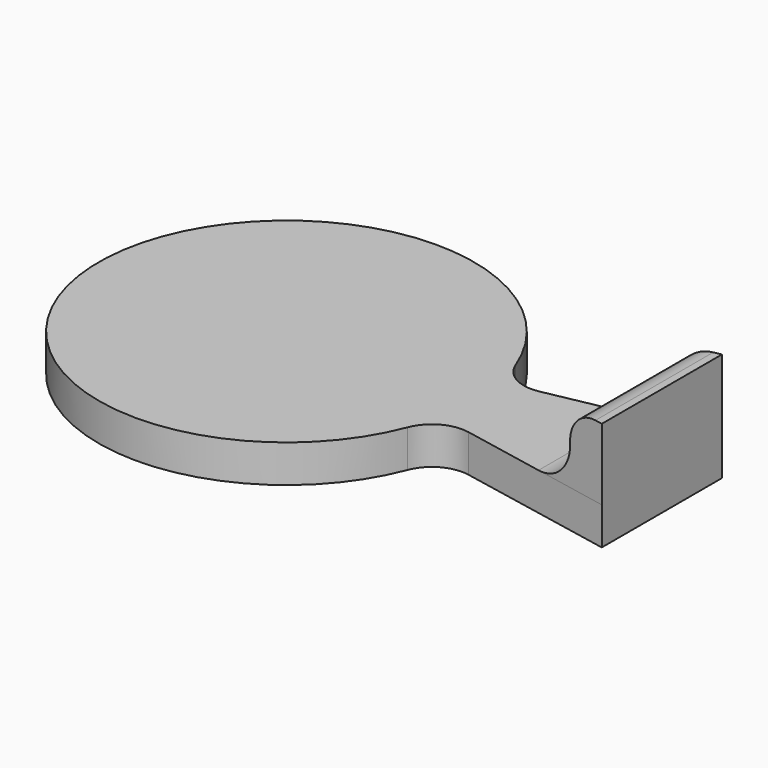
from build123d import *

# Parameters (mm, degrees)
F1_DEPTH = 5
F3_DEPTH = 9.5
F4_R     = 5
F5_R     = 4


# Not quite as in the source:
# - a feature names something its author has since deleted; it is built from what else it names


with BuildPart() as f1:
    # F0 (on Top) → F1 (new body)
    with BuildSketch(Plane.XY):
        with BuildLine():
            Line((50, 10), (24.4948974278, 5))
            ThreePointArc((24.4948974278, 5), (-25, 0), (24.4948974278, -5))
            Line((24.4948974278, -5), (50, -10))
            Line((50, -10), (50, 10))
        make_face()
    extrude(amount=F1_DEPTH)

    # F2 (on face) → F3 (join)
    with BuildSketch(Plane.XY.offset(5)):
        Polygon((50, -10), (50, 10), (45, 9.0198039812), (45, -9.0198039812), align=None)
    extrude(amount=F3_DEPTH)

    # F4
    f4_edges = [f1.edges().sort_by_distance(p)[0] for p in [
        (45, 0, 5),
        (24.494897, -5, 2.5),
        (24.494897, 5, 2.5),
    ]]
    fillet(f4_edges, radius=F4_R)

    # F5
    f5_edges = [f1.edges().sort_by_distance(p)[0] for p in [
        (45, 0, 14.5),
    ]]
    fillet(f5_edges, radius=F5_R)


solid = f1.part
